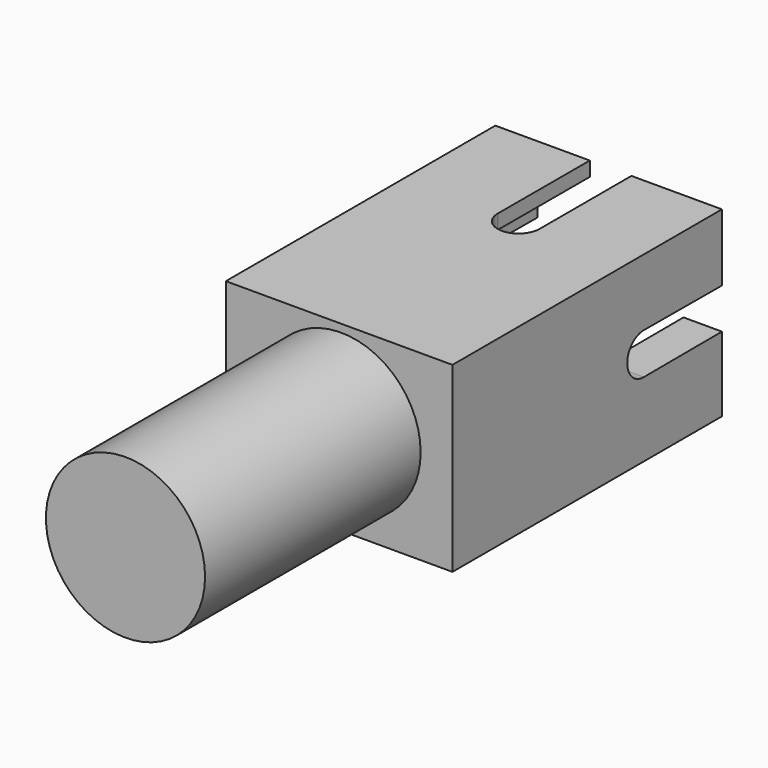
from build123d import *

# Parameters (mm, degrees)
F0_R     = 6
F1_DEPTH = 20.32
F2_W     = 17.0879438519
F2_H     = 13.7446504086
F3_DEPTH = 25.4
F5_DEPTH = 11.43
F7_DEPTH = 25.4
F9_DEPTH = 25.4


# Not quite as in the source:
# - a feature names something its author has since deleted; it is built from what else it names


with BuildPart() as f1:
    # F0 (on Front) → F1 (new body)
    with BuildSketch(Plane.XZ):
        Circle(F0_R)
    extrude(amount=F1_DEPTH)

    # F2 (on face) → F3 (join)
    with BuildSketch(Plane(origin=(0, 0, 0), x_dir=(-1, 0, 0), z_dir=(0, 1, 0))):
        with Locations((0.1456169412, -0.2847756259)):
            Rectangle(F2_W, F2_H)
    extrude(amount=F3_DEPTH)

    # F4 (on face) → F5 (cut)
    with BuildSketch(Plane(origin=(0, 25.4, 0), x_dir=(-1, 0, 0), z_dir=(0, 1, 0))):
        Polygon((5.5, 5.5), (0, 5.5), (-5.5, 5.5), (-5.5, -5.5), (5.5, -5.5), align=None)
    extrude(amount=-F5_DEPTH, mode=Mode.SUBTRACT)

    # F6 (on face) → F7 (cut)
    with BuildSketch(Plane(origin=(0, 0, -7.1571008302), x_dir=(1, 0, 0), z_dir=(0, 0, -1))):
        with BuildLine():
            Line((1.5748, -25.4), (1.5748, -16.734668985))
            ThreePointArc((1.5748, -16.734668985), (0, -15.159868985), (-1.5748, -16.734668985))
            ThreePointArc((-1.5748, -16.734668985), (-1.574798986, -16.7364561088), (-1.5747959439, -16.7382432303))
            Line((-1.5747959439, -16.7382432303), (-1.5649663519, -25.4))
            Line((-1.5649663519, -25.4), (1.5748, -25.4))
        make_face()
    extrude(amount=-F7_DEPTH, mode=Mode.SUBTRACT)

    # F8 (on face) → F9 (cut)
    with BuildSketch(Plane(origin=(-8.6895888671, 0, 0), x_dir=(0, -1, 0), z_dir=(-1, 0, 0))):
        with BuildLine():
            Line((-25.4, -1.5290330871), (-18.0435866661, -1.5568010835))
            ThreePointArc((-18.0435866661, -1.5568010835), (-18.0377102216, -1.5568343561), (-18.0318336934, -1.556845447))
            ThreePointArc((-18.0318336934, -1.556845447), (-16.4749882464, 0), (-18.0318336934, 1.556845447))
            ThreePointArc((-18.0318336934, 1.556845447), (-18.0377102216, 1.5568343561), (-18.0435866661, 1.5568010835))
            Line((-18.0435866661, 1.5568010835), (-25.4, 1.5290330871))
            Line((-25.4, 1.5290330871), (-25.4, -1.5290330871))
        make_face()
    extrude(amount=-F9_DEPTH, mode=Mode.SUBTRACT)


solid = f1.part
